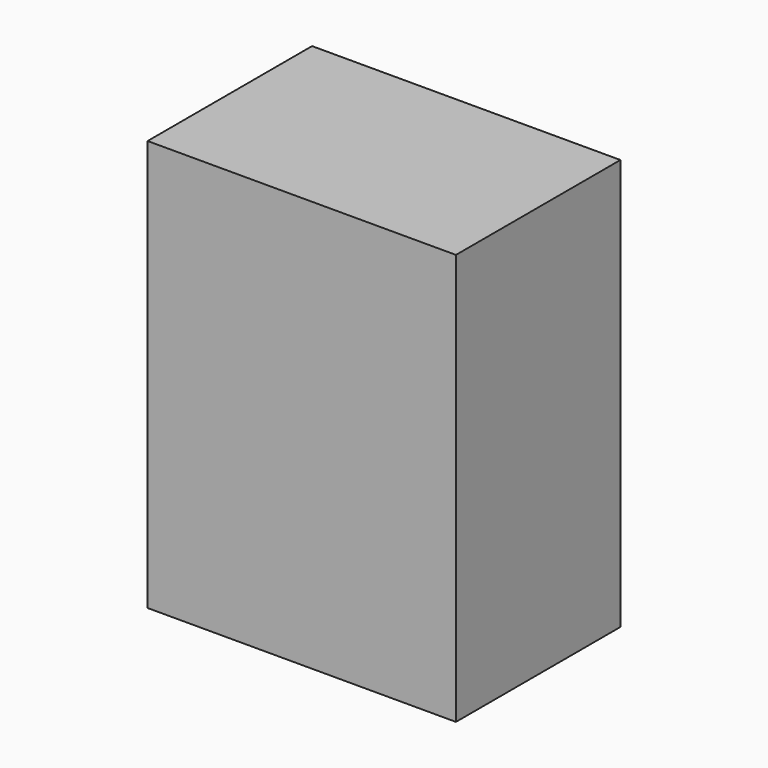
from build123d import *

# Parameters (mm, degrees)
F0_W     = 25.4
F0_H     = 50.8
F1_DEPTH = 25.4
F2_ANGLE = 90
F3_DEPTH = 12.7


# Not quite as in the source:
# - the program builds the solid bodies; features that only make, move or delete a surface that nothing else refers to are left out


with BuildPart() as f1:
    # F0 (on Top) → F1 (new body)
    with BuildSketch(Plane.XY):
        with Locations((12.7, 25.4)):
            Rectangle(F0_W, F0_H)
    extrude(amount=F1_DEPTH)


with BuildPart() as f1_1:
    # F2: moved
    add(f1.part.rotate(Axis((12.7, 0, 0), (1, 0, 0)), F2_ANGLE))

    # F3 (add): a face of the model
    f3_faces = [f1_1.faces().sort_by_distance(p)[0] for p in [
        (0, -12.7, 25.4),
    ]]
    extrude(f3_faces, amount=F3_DEPTH)


with BuildPart() as f1_2:
    # F5: moved
    add(f1_1.part.moved(Location((-6.35, 0, 0))))


solid = f1_2.part
